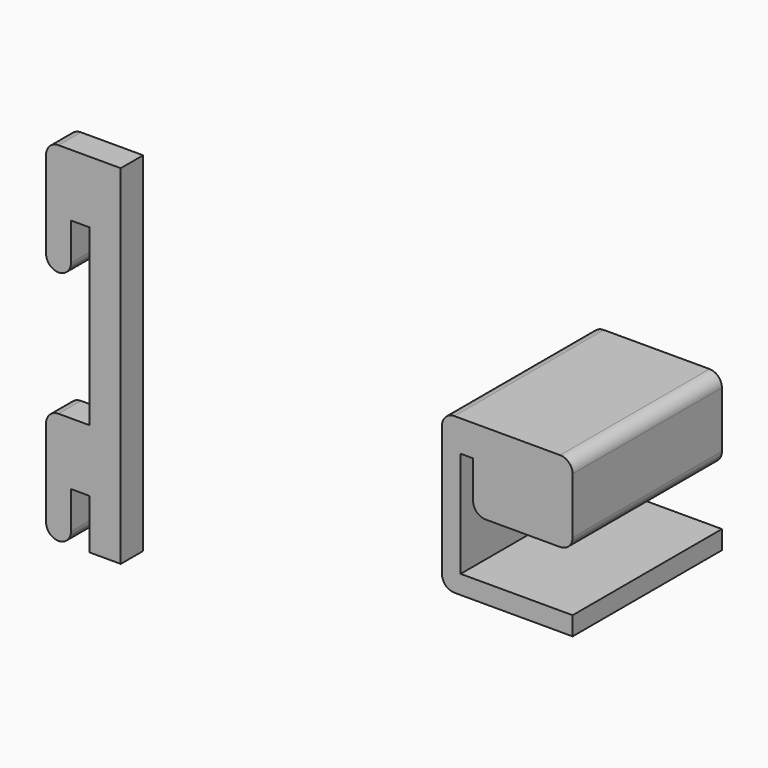
from build123d import *

# Parameters (mm, degrees)
F1_DEPTH = 30
F2_R     = 2
F3_W     = 3
F3_H     = 10
F4_DEPTH = 4.5
F6_R     = 1.99999


# Not quite as in the source:
# - a fillet or chamfer is up to 0.001 mm smaller than in the source, because OpenCascade refuses the exact size


with BuildPart() as f1:
    # F0 (on Front) → F1 (new body)
    with BuildSketch(Plane.XZ):
        Polygon((5, 12), (21, 12), (21, 25), (0, 25), (0, 0), (21, 0), (21, 3), (3, 3), (3, 20), (5, 20), align=None)
    extrude(amount=-F1_DEPTH)

    # F2
    f2_edges = [f1.edges().sort_by_distance(p)[0] for p in [
        (21, 15, 25),
        (0, 15, 25),
        (21, 15, 12),
        (0, 15, 0),
        (5, 15, 12),
    ]]
    fillet(f2_edges, radius=F2_R)


with BuildPart() as f4:
    # F3 (on Front) → F4 (new body)
    with BuildSketch(Plane.XZ):
        Polygon((-56.0359997153, 45.6349952309), (-60.0359997153, 45.6349952309), (-60.0359997153, 27.6349952309), (-56.0359997153, 27.6349952309), (-56.0359997153, 35.6349952309), align=None)
        with Locations((-54.5359997153, 40.6349952309)):
            Rectangle(F3_W, F3_H)
        Polygon((-48.0359997153, 45.6349952309), (-53.0359997153, 45.6349952309), (-53.0359997153, 35.6349952309), (-53.0359997153, 7.6349952309), (-53.0359997153, -2.3650047691), (-53.0359997153, -10.3650047691), (-48.0359997153, -10.3650047691), align=None)
        with Locations((-54.5359997153, 2.6349952309)):
            Rectangle(F3_W, F3_H)
        Polygon((-56.0359997153, -2.3650047691), (-56.0359997153, 7.6349952309), (-60.0359997153, 7.6349952309), (-60.0359997153, -10.3650047691), (-56.0359997153, -10.3650047691), align=None)
    extrude(amount=F4_DEPTH)

    # F6 (radius 2 in the source; OpenCascade refuses exactly that, so slightly less here)
    f6_edges = [f4.edges().sort_by_distance(p)[0] for p in [
        (-56.036, -2.25, -10.365005),
        (-60.036, -2.25, -10.365005),
        (-60.036, -2.25, 7.634995),
        (-60.036, -2.25, 27.634995),
        (-56.036, -2.25, 27.634995),
        (-60.036, -2.25, 45.634995),
    ]]
    fillet(f6_edges, radius=F6_R)


solid = Compound([f1.part, f4.part])
